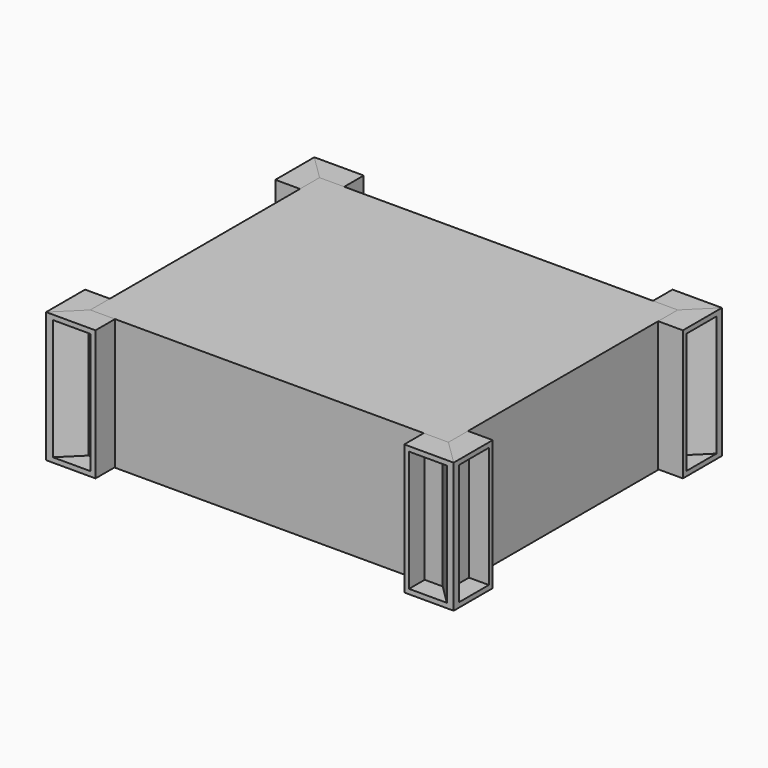
from build123d import *

# Parameters (mm, degrees)
F0_W     = 5.1724143326
F0_H     = 5.1077616215
F1_DEPTH = 27.4
F2_DEPTH = 27.3
F3_DEPTH = 27.3
F4_T     = -1
F4_2_T   = -1
F4_3_T   = -1
F4_4_T   = -1
F4_5_T   = -1
F4_6_T   = -1
F4_7_T   = -1
F4_8_T   = -1


# Not quite as in the source:
# - the program builds the solid bodies; features that only make, move or delete a surface that nothing else refers to are left out


with BuildPart() as f1:
    # F0 (on Top) → F1 (new body)
    with BuildSketch(Plane.XY):
        Polygon((-32.3275856674, -30), (32.3275856674, -30), (32.3275856674, -24.8922383785), (37.5, -24.8922383785), (37.5, 24.8922383785), (32.3275856674, 24.8922383785), (32.3275856674, 30), (-32.3275856674, 30), (-32.3275856674, 24.8922383785), (-37.5, 24.8922383785), (-37.5, -24.8922383785), (-32.3275856674, -24.8922383785), align=None)
        with Locations((-34.9137928337, 27.4461191893)):
            Rectangle(F0_W, F0_H)
        with Locations((34.9137928337, 27.4461191893)):
            Rectangle(F0_W, F0_H)
        with Locations((34.9137928337, -27.4461191893)):
            Rectangle(F0_W, F0_H)
        with Locations((-34.9137928337, -27.4461191893)):
            Rectangle(F0_W, F0_H)
    extrude(amount=-F1_DEPTH)


with BuildPart() as f2:
    # F0 (on Top) → F2 (new body)
    with BuildSketch(Plane.XY):
        Polygon((-42.6724143326, 24.8922383785), (-37.5, 24.8922383785), (-37.5, 30), (-42.6724143326, 35.1077616215), align=None)
    extrude(amount=-F2_DEPTH)

    # F4#7
    f4_7_openings = [f2.faces().sort_by_distance(p)[0] for p in [
        (-42.672414, 30, -13.65),
    ]]
    offset(amount=F4_7_T, openings=f4_7_openings)


with BuildPart() as f2b:
    # F0 (on Top) → F2, piece 2 (new body)
    with BuildSketch(Plane.XY):
        Polygon((32.3275856674, 30), (37.5, 30), (42.6724143326, 35.1077616215), (32.3275856674, 35.1077616215), align=None)
    extrude(amount=-F2_DEPTH)

    # F4#3
    f4_3_openings = [f2b.faces().sort_by_distance(p)[0] for p in [
        (37.5, 35.107762, -13.65),
    ]]
    offset(amount=F4_3_T, openings=f4_3_openings)


with BuildPart() as f2c:
    # F0 (on Top) → F2, piece 3 (new body)
    with BuildSketch(Plane.XY):
        Polygon((37.5, -24.8922383785), (37.5, -30), (42.6724143326, -35.1077616215), (42.6724143326, -24.8922383785), align=None)
    extrude(amount=-F2_DEPTH)

    # F4
    f4_openings = [f2c.faces().sort_by_distance(p)[0] for p in [
        (42.672414, -30, -13.65),
    ]]
    offset(amount=F4_T, openings=f4_openings, kind=Kind.INTERSECTION)


with BuildPart() as f2d:
    # F0 (on Top) → F2, piece 4 (new body)
    with BuildSketch(Plane.XY):
        Polygon((-42.6724143326, -35.1077616215), (-37.5, -30), (-37.5, -24.8922383785), (-42.6724143326, -24.8922383785), align=None)
    extrude(amount=-F2_DEPTH)

    # F4#5
    f4_5_openings = [f2d.faces().sort_by_distance(p)[0] for p in [
        (-42.672414, -30, -13.65),
    ]]
    offset(amount=F4_5_T, openings=f4_5_openings)


with BuildPart() as f3:
    # F0 (on Top) → F3 (new body)
    with BuildSketch(Plane.XY):
        Polygon((-37.5, 30), (-32.3275856674, 30), (-32.3275856674, 35.1077616215), (-42.6724143326, 35.1077616215), align=None)
    extrude(amount=-F3_DEPTH)

    # F4#4
    f4_4_openings = [f3.faces().sort_by_distance(p)[0] for p in [
        (-37.5, 35.107762, -13.65),
    ]]
    offset(amount=F4_4_T, openings=f4_4_openings)


with BuildPart() as f3b:
    # F0 (on Top) → F3, piece 2 (new body)
    with BuildSketch(Plane.XY):
        Polygon((37.5, 30), (37.5, 24.8922383785), (42.6724143326, 24.8922383785), (42.6724143326, 35.1077616215), align=None)
    extrude(amount=-F3_DEPTH)

    # F4#2
    f4_2_openings = [f3b.faces().sort_by_distance(p)[0] for p in [
        (42.672414, 30, -13.65),
    ]]
    offset(amount=F4_2_T, openings=f4_2_openings)


with BuildPart() as f3c:
    # F0 (on Top) → F3, piece 3 (new body)
    with BuildSketch(Plane.XY):
        Polygon((42.6724143326, -35.1077616215), (37.5, -30), (32.3275856674, -30), (32.3275856674, -35.1077616215), align=None)
    extrude(amount=-F3_DEPTH)

    # F4#8
    f4_8_openings = [f3c.faces().sort_by_distance(p)[0] for p in [
        (37.5, -35.107762, -13.65),
    ]]
    offset(amount=F4_8_T, openings=f4_8_openings)


with BuildPart() as f3d:
    # F0 (on Top) → F3, piece 4 (new body)
    with BuildSketch(Plane.XY):
        Polygon((-32.3275856674, -35.1077616215), (-32.3275856674, -30), (-37.5, -30), (-42.6724143326, -35.1077616215), align=None)
    extrude(amount=-F3_DEPTH)

    # F4#6
    f4_6_openings = [f3d.faces().sort_by_distance(p)[0] for p in [
        (-37.5, -35.107762, -13.65),
    ]]
    offset(amount=F4_6_T, openings=f4_6_openings)


solid = Compound([f1.part, f2.part, f2b.part, f2c.part, f2d.part, f3.part, f3b.part, f3c.part, f3d.part])
